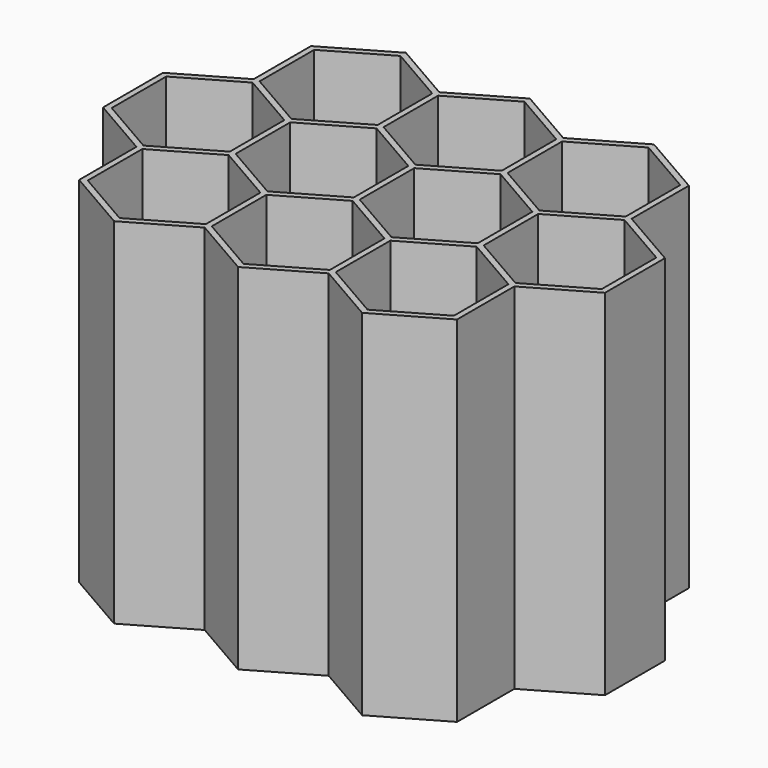
from build123d import *

# Parameters (mm, degrees)
F2_DEPTH = 90


with BuildPart() as f2:
    # F0 (on Top) → F2 (new body)
    with BuildSketch(Plane.XY):
        Polygon((0.75, 17.7535207776), (0, 17.3205080757), (15, 8.6602540378), (15, 9.5262794416), (15.75, 9.9592921435), (0.75, 18.6195461814), align=None)
        Polygon((-0.75, 17.7535207776), (0, 17.3205080757), (0.75, 17.7535207776), (0.75, 18.6195461814), (0, 19.0525588833), (-0.75, 18.6195461814), align=None)
        Polygon((-15, 8.6602540378), (0, 17.3205080757), (-0.75, 17.7535207776), (-0.75, 18.6195461814), (-15.75, 9.9592921435), (-16.5, 9.5262794416), (-16.5, 8.6602540378), (-15.75, 8.227241336), align=None)
        Polygon((15.75, 8.227241336), (15, 8.6602540378), (15, -8.6602540378), (15, -9.5262794416), (15.75, -9.9592921435), (16.5, -9.5262794416), (16.5, -8.6602540378), (16.5, 8.6602540378), align=None)
        Polygon((15, 9.5262794416), (15, 8.6602540378), (15.75, 8.227241336), (16.5, 8.6602540378), (16.5, 9.5262794416), (15.75, 9.9592921435), align=None)
        Polygon((-15, -8.6602540378), (-15, 8.6602540378), (-15.75, 8.227241336), (-16.5, 8.6602540378), (-16.5, -9.5262794416), (0, -19.0525588833), (15.75, -9.9592921435), (15, -9.5262794416), (15, -8.6602540378), (0, -17.3205080757), align=None)
        Polygon((0, 19.0525588833), (0.75, 18.6195461814), (0.75, 35.9400542571), (0, 35.5070415552), (-0.75, 35.9400542571), (-0.75, 18.6195461814), align=None)
        Polygon((30.75, 18.6195461814), (15.75, 9.9592921435), (16.5, 9.5262794416), (16.5, 8.6602540378), (31.5, 17.3205080757), (30.75, 17.7535207776), align=None)
        Polygon((-32.25, 17.7535207776), (-16.5, 8.6602540378), (-16.5, 9.5262794416), (-15.75, 9.9592921435), (-30.75, 18.6195461814), (-30.75, 35.9400542571), (-15.75, 44.6003082949), (-16.5, 45.0333209968), (-16.5, 45.8993464006), (-32.25, 36.8060796608), align=None)
        Polygon((0, 35.5070415552), (0.75, 35.9400542571), (0.75, 36.8060796608), (0, 37.2390923627), (-0.75, 36.8060796608), (-0.75, 35.9400542571), align=None)
        Polygon((0.75, 36.8060796608), (0.75, 35.9400542571), (15.75, 44.6003082949), (15, 45.0333209968), (15, 45.8993464006), (0, 37.2390923627), align=None)
        Polygon((-15.75, 44.6003082949), (-0.75, 35.9400542571), (-0.75, 36.8060796608), (0, 37.2390923627), (-15, 45.8993464006), (-15.75, 46.3323591025), (-16.5, 45.8993464006), (-16.5, 45.0333209968), align=None)
        Polygon((16.5, -9.5262794416), (15.75, -9.9592921435), (31.5, -19.0525588833), (47.25, -9.9592921435), (46.5, -9.5262794416), (46.5, -8.6602540378), (31.5, -17.3205080757), (16.5, -8.6602540378), align=None)
        Polygon((30.75, 35.9400542571), (30.75, 18.6195461814), (31.5, 19.0525588833), (32.25, 18.6195461814), (32.25, 35.9400542571), (31.5, 35.5070415552), align=None)
        Polygon((31.5, 19.0525588833), (30.75, 18.6195461814), (30.75, 17.7535207776), (31.5, 17.3205080757), (32.25, 17.7535207776), (32.25, 18.6195461814), align=None)
        Polygon((32.25, 17.7535207776), (31.5, 17.3205080757), (46.5, 8.6602540378), (46.5, 9.5262794416), (47.25, 9.9592921435), (32.25, 18.6195461814), align=None)
        Polygon((16.5, 45.0333209968), (15.75, 44.6003082949), (30.75, 35.9400542571), (30.75, 36.8060796608), (31.5, 37.2390923627), (16.5, 45.8993464006), align=None)
        Polygon((15, 45.0333209968), (15.75, 44.6003082949), (16.5, 45.0333209968), (16.5, 45.8993464006), (15.75, 46.3323591025), (15, 45.8993464006), align=None)
        Polygon((30.75, 36.8060796608), (30.75, 35.9400542571), (31.5, 35.5070415552), (32.25, 35.9400542571), (32.25, 36.8060796608), (31.5, 37.2390923627), align=None)
        Polygon((47.25, 8.227241336), (46.5, 8.6602540378), (46.5, -8.6602540378), (46.5, -9.5262794416), (47.25, -9.9592921435), (48, -9.5262794416), (48, -8.6602540378), (48, 8.6602540378), align=None)
        Polygon((46.5, 9.5262794416), (46.5, 8.6602540378), (47.25, 8.227241336), (48, 8.6602540378), (48, 9.5262794416), (47.25, 9.9592921435), align=None)
        Polygon((48, -9.5262794416), (47.25, -9.9592921435), (63, -19.0525588833), (79.5, -9.5262794416), (79.5, 8.6602540378), (78.75, 8.227241336), (78, 8.6602540378), (78, -8.6602540378), (63, -17.3205080757), (48, -8.6602540378), align=None)
        Polygon((-16.5, 64.08587988), (-16.5, 45.8993464006), (-15.75, 46.3323591025), (-15, 45.8993464006), (-15, 63.2198544763), (0, 71.8801085141), (15, 63.2198544763), (15, 64.08587988), (15.75, 64.5188925819), (0, 73.6121593217), align=None)
        Polygon((15, 63.2198544763), (15, 45.8993464006), (15.75, 46.3323591025), (16.5, 45.8993464006), (16.5, 63.2198544763), (16.5, 64.08587988), (15.75, 64.5188925819), (15, 64.08587988), align=None)
        Polygon((62.25, 18.6195461814), (47.25, 9.9592921435), (48, 9.5262794416), (48, 8.6602540378), (63, 17.3205080757), (62.25, 17.7535207776), align=None)
        Polygon((32.25, 36.8060796608), (32.25, 35.9400542571), (47.25, 44.6003082949), (46.5, 45.0333209968), (46.5, 45.8993464006), (31.5, 37.2390923627), align=None)
        Polygon((16.5, 64.08587988), (16.5, 63.2198544763), (31.5, 71.8801085141), (46.5, 63.2198544763), (46.5, 64.08587988), (47.25, 64.5188925819), (31.5, 73.6121593217), (15.75, 64.5188925819), align=None)
        Polygon((62.25, 35.9400542571), (62.25, 18.6195461814), (63, 19.0525588833), (63.75, 18.6195461814), (63.75, 35.9400542571), (63, 35.5070415552), align=None)
        Polygon((63, 19.0525588833), (62.25, 18.6195461814), (62.25, 17.7535207776), (63, 17.3205080757), (63.75, 17.7535207776), (63.75, 18.6195461814), align=None)
        Polygon((48, 45.0333209968), (47.25, 44.6003082949), (62.25, 35.9400542571), (62.25, 36.8060796608), (63, 37.2390923627), (48, 45.8993464006), align=None)
        Polygon((46.5, 45.0333209968), (47.25, 44.6003082949), (48, 45.0333209968), (48, 45.8993464006), (47.25, 46.3323591025), (46.5, 45.8993464006), align=None)
        Polygon((46.5, 63.2198544763), (46.5, 45.8993464006), (47.25, 46.3323591025), (48, 45.8993464006), (48, 63.2198544763), (48, 64.08587988), (47.25, 64.5188925819), (46.5, 64.08587988), align=None)
        Polygon((63.75, 17.7535207776), (63, 17.3205080757), (78, 8.6602540378), (78.75, 8.227241336), (79.5, 8.6602540378), (79.5, 9.5262794416), (78.75, 9.9592921435), (63.75, 18.6195461814), align=None)
        Polygon((79.5, 9.5262794416), (79.5, 8.6602540378), (95.25, 17.7535207776), (95.25, 36.8060796608), (79.5, 45.8993464006), (79.5, 45.0333209968), (78.75, 44.6003082949), (93.75, 35.9400542571), (93.75, 18.6195461814), (78.75, 9.9592921435), align=None)
        Polygon((62.25, 36.8060796608), (62.25, 35.9400542571), (63, 35.5070415552), (63.75, 35.9400542571), (63.75, 36.8060796608), (63, 37.2390923627), align=None)
        Polygon((63.75, 36.8060796608), (63.75, 35.9400542571), (78.75, 44.6003082949), (79.5, 45.0333209968), (79.5, 45.8993464006), (78.75, 46.3323591025), (78, 45.8993464006), (63, 37.2390923627), align=None)
        Polygon((48, 64.08587988), (48, 63.2198544763), (63, 71.8801085141), (78, 63.2198544763), (78, 45.8993464006), (78.75, 46.3323591025), (79.5, 45.8993464006), (79.5, 64.08587988), (63, 73.6121593217), (47.25, 64.5188925819), align=None)
    extrude(amount=F2_DEPTH)


solid = f2.part
